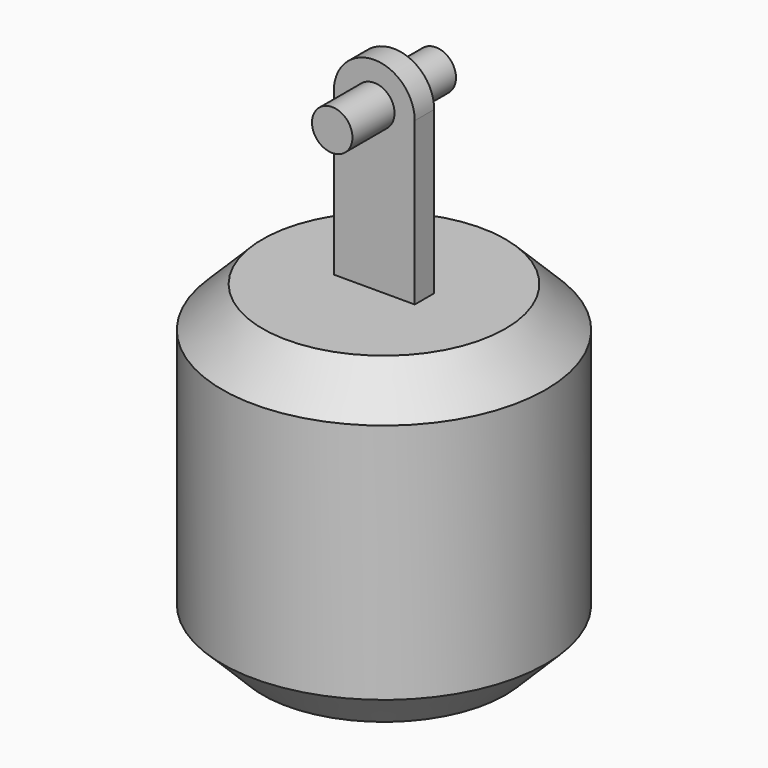
from build123d import *

# Parameters (mm, degrees)
F0_R     = 2.5
F1_DEPTH = 8
F3_DEPTH = 1.5
F4_R     = 20
F5_DEPTH = 39.84388
F6_SIZE  = 5


with BuildPart() as f1:
    # F0 (on Front) → F1 (new body, symmetric)
    with BuildSketch(Plane.XZ):
        Circle(F0_R)
    extrude(amount=F1_DEPTH, both=True)

    # F2 (on Front) → F3 (join, symmetric)
    with BuildSketch(Plane.XZ):
        with BuildLine():
            ThreePointArc((5, 0), (0, 5), (-5, 0))
            Line((-5, 0), (-5, -20))
            Line((-5, -20), (5, -20))
            Line((5, -20), (5, 0))
        make_face()
    extrude(amount=F3_DEPTH, both=True)

    # F4 (on face) → F5 (join)
    with BuildSketch(Plane(origin=(0, 0, -20), x_dir=(1, 0, 0), z_dir=(0, 0, -1))):
        Circle(F4_R)
    extrude(amount=F5_DEPTH)

    # F6
    f6_edges = [f1.edges().sort_by_distance(p)[0] for p in [
        (-20, 0, -20),
        (-20, 0, -59.84388),
    ]]
    chamfer(f6_edges, length=F6_SIZE)


solid = f1.part
